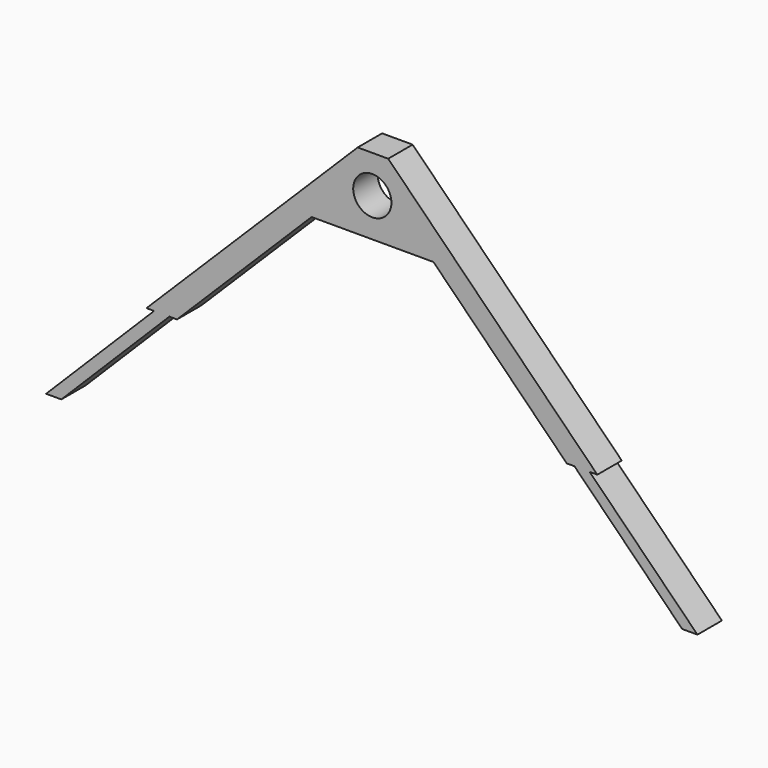
from build123d import *

# Parameters (mm, degrees)
F0_R     = 6.35
F1_DEPTH = 10.16


# Not quite as in the source:
# - a feature names something its author has since deleted; it is built from what else it names


with BuildPart() as f1:
    # F0 (on Front) → F1 (new body)
    with BuildSketch(Plane.XZ):
        Polygon((-4.8744329511, 71.2045607365), (-75.0909721843, 1.3295207142), (-72.5509721843, 1.3295207142), (-108.4719966685, -34.5915037701), (-103.3919966685, -34.5915037701), (-67.4709721843, 1.3295207142), (-64.9309721843, 1.3295207142), (-20.1762745117, 45.8665532311), (-4.9362745117, 45.8665532311), (5.2855670489, 45.8665532311), (20.3403427678, 45.8665532311), (64.660768747, 1.3295207142), (67.200768747, 1.3295207142), (103.0377074058, -34.6753932222), (108.1177074058, -34.6753932222), (72.2719103919, 1.3207015165), (74.820768747, 1.3295207142), (5.2855670489, 71.2045607365), align=None)
        with Locations((0, 58.6755184585)):
            Circle(F0_R, mode=Mode.SUBTRACT)
    extrude(amount=F1_DEPTH)


solid = f1.part
